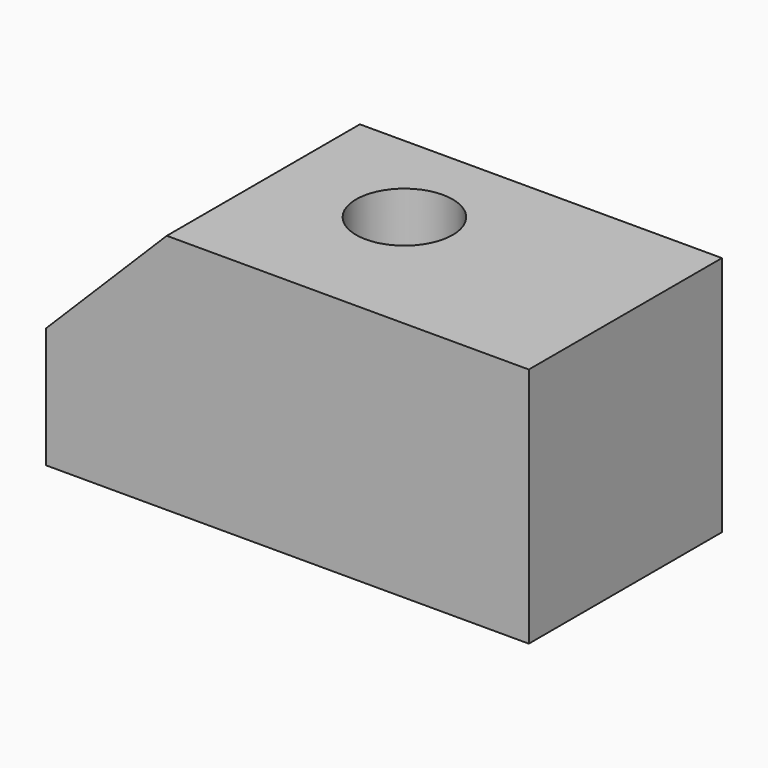
from build123d import *

# Parameters (mm, degrees)
F0_W     = 304.8
F0_H     = 152.4
F1_DEPTH = 152.4
F9_R     = 30.48
F5_DEPTH = 152.401
F6_SIZE  = 76.2
F8_DEPTH = 30.48


# Not quite as in the source:
# - the program builds the solid bodies; features that only make, move or delete a surface that nothing else refers to are left out


with BuildPart() as f1:
    # F0 (on Top) → F1 (new body)
    with BuildSketch(Plane.XY):
        with Locations((-2.8575006872, -27.8319329938)):
            Rectangle(F0_W, F0_H)
    extrude(amount=F1_DEPTH)

    # F9 (on face) → F5 (cut, through all)
    with BuildSketch(Plane.XY.offset(152.4)):
        with Locations((0, -15.3043069538)):
            Circle(F9_R)
    extrude(amount=-F5_DEPTH, mode=Mode.SUBTRACT)

    # F6
    f6_edges = [f1.edges().sort_by_distance(p)[0] for p in [
        (-155.257501, -27.831933, 152.4),
    ]]
    chamfer(f6_edges, length=F6_SIZE)

    # F7 (on face) → F8 (cut)
    with BuildSketch(Plane(origin=(0, 0, 0), x_dir=(1, 0, 0), z_dir=(0, 0, -1))):
        with BuildLine():
            ThreePointArc((-124.6516630054, 78.40236485), (-134.6516630054, 68.40236485), (-124.6516630054, 58.40236485))
            Line((-124.6516630054, 58.40236485), (-75.9895667434, 58.40236485))
            ThreePointArc((-75.9895667434, 58.40236485), (-65.9895667434, 68.40236485), (-75.9895667434, 78.40236485))
            Line((-75.9895667434, 78.40236485), (-124.6516630054, 78.40236485))
        make_face()
    extrude(amount=-F8_DEPTH, mode=Mode.SUBTRACT)


solid = f1.part
